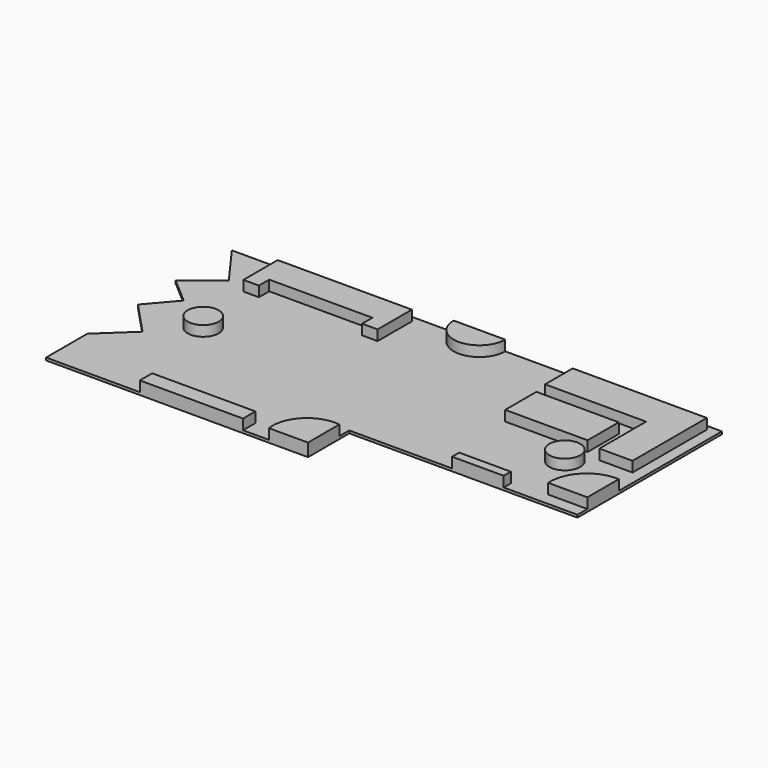
from build123d import *

# Parameters (mm, degrees)
F0_W      = 5077.0874023438
F0_H      = 1000
F1_DEPTH  = 50
F2_W      = 300
F2_H      = 250
F2_W_2    = 1596.8501567841
F2_H_2    = 755.4990053177
F2_W_3    = 1000
F2_H_3    = 172.0993051472
F2_W_4    = 2000
F2_H_4    = 300
F2_R      = 300
F3_DEPTH  = 200
F4_DEPTH  = 200
F5_DEPTH  = 200
F6_DEPTH  = 200
F7_DEPTH  = 200
F8_DEPTH  = 200
F10_DEPTH = 25


# Not quite as in the source:
# - the program builds the solid bodies; features that only make, move or delete a surface that nothing else refers to are left out


with BuildPart() as f1:
    # F0 (on Top) → F1 (new body)
    with BuildSketch(Plane.XY):
        Polygon((-777.0874023438, 2275.4955291748), (-5077.0874023438, 2275.4955291748), (-4499.191295666, 1480.7769234966), (-5119.9254926672, 968.8577861197), (-4616.2895248949, 535.3893431642), (-5077.0874023438, 0), (-4466.0972264549, -651.5435160618), (-5077.0874023438, -1224.5044708252), (0, -1224.5044708252), (4422.9125976562, -1224.5044708252), (4422.9125976562, 2275.4955291748), (222.9125976562, 2275.4955291748), align=None)
        with Locations((-2538.5437011719, -1724.5044708252)):
            Rectangle(F0_W, F0_H)
    extrude(amount=F1_DEPTH)

    # F2 (on face) → F3 (join)
    with BuildSketch(Plane.XY.offset(50)):
        Polygon((-1494.8213815689, 2159.7741413116), (-4094.8213815689, 2159.7741413116), (-4094.8213815689, 1579.7741413116), (-3794.8213815689, 1579.7741413116), (-1794.8213815689, 1579.7741413116), (-1494.8213815689, 1579.7741413116), align=None)
        with Locations((-3944.8213815689, 1454.7741413116)):
            Rectangle(F2_W, F2_H)
        with Locations((-1644.8213815689, 1454.7741413116)):
            Rectangle(F2_W, F2_H)
        Polygon((4209.393954277, 2177.0670413971), (1609.393954277, 2177.0670413971), (1609.393954277, 1507.4201822281), (3566.8230056763, 1507.4201822281), (3566.8230056763, 377.0670413971), (4209.393954277, 377.0670413971), align=None)
        with Locations((2459.3304395676, 854.9439311028)):
            Rectangle(F2_W_2, F2_H_2)
        with Locations((2492.1946525574, -1138.4548182516)):
            Rectangle(F2_W_3, F2_H_3)
        with BuildLine():
            Line((222.9125976562, 2275.4955291748), (-777.0874023438, 2275.4955291748))
            ThreePointArc((-777.0874023438, 2275.4955291748), (-277.0874023438, 1775.4955291748), (222.9125976562, 2275.4955291748))
        make_face()
        with BuildLine():
            Line((3662.9125976562, -984.1235280037), (4422.9125976562, -984.1235280037))
            Line((4422.9125976562, -984.1235280037), (4422.9125976562, -224.1235280037))
            ThreePointArc((4422.9125976562, -224.1235280037), (3868.7706575404, -429.9815878879), (3662.9125976562, -984.1235280037))
        make_face()
        with Locations((-2260, -2074.5044708252)):
            Rectangle(F2_W_4, F2_H_4)
        with BuildLine():
            Line((-760, -2224.5044708252), (0, -2224.5044708252))
            Line((0, -2224.5044708252), (0, -1464.5044708252))
            ThreePointArc((0, -1464.5044708252), (-569.1431166961, -1655.361354129), (-760, -2224.5044708252))
        make_face()
        with Locations((-3832.0874023438, 25.4955291748)):
            Circle(F2_R)
        with Locations((3177.9125976562, 25.4955291748)):
            Circle(F2_R)
    extrude(amount=F3_DEPTH)

    # F2 (on face) → F4 (join)
    with BuildSketch(Plane.XY.offset(50)):
        Polygon((-1494.8213815689, 2159.7741413116), (-4094.8213815689, 2159.7741413116), (-4094.8213815689, 1579.7741413116), (-3794.8213815689, 1579.7741413116), (-1794.8213815689, 1579.7741413116), (-1494.8213815689, 1579.7741413116), align=None)
        with Locations((-3944.8213815689, 1454.7741413116)):
            Rectangle(F2_W, F2_H)
        with Locations((-1644.8213815689, 1454.7741413116)):
            Rectangle(F2_W, F2_H)
        Polygon((4209.393954277, 2177.0670413971), (1609.393954277, 2177.0670413971), (1609.393954277, 1507.4201822281), (3566.8230056763, 1507.4201822281), (3566.8230056763, 377.0670413971), (4209.393954277, 377.0670413971), align=None)
        with Locations((2459.3304395676, 854.9439311028)):
            Rectangle(F2_W_2, F2_H_2)
        with Locations((2492.1946525574, -1138.4548182516)):
            Rectangle(F2_W_3, F2_H_3)
        with BuildLine():
            Line((222.9125976562, 2275.4955291748), (-777.0874023438, 2275.4955291748))
            ThreePointArc((-777.0874023438, 2275.4955291748), (-277.0874023438, 1775.4955291748), (222.9125976562, 2275.4955291748))
        make_face()
        with BuildLine():
            Line((3662.9125976562, -984.1235280037), (4422.9125976562, -984.1235280037))
            Line((4422.9125976562, -984.1235280037), (4422.9125976562, -224.1235280037))
            ThreePointArc((4422.9125976562, -224.1235280037), (3868.7706575404, -429.9815878879), (3662.9125976562, -984.1235280037))
        make_face()
        with Locations((-2260, -2074.5044708252)):
            Rectangle(F2_W_4, F2_H_4)
        with BuildLine():
            Line((-760, -2224.5044708252), (0, -2224.5044708252))
            Line((0, -2224.5044708252), (0, -1464.5044708252))
            ThreePointArc((0, -1464.5044708252), (-569.1431166961, -1655.361354129), (-760, -2224.5044708252))
        make_face()
        with Locations((-3832.0874023438, 25.4955291748)):
            Circle(F2_R)
        with Locations((3177.9125976562, 25.4955291748)):
            Circle(F2_R)
    extrude(amount=F4_DEPTH)

    # F2 (on face) → F5 (join)
    with BuildSketch(Plane.XY.offset(50)):
        Polygon((-1494.8213815689, 2159.7741413116), (-4094.8213815689, 2159.7741413116), (-4094.8213815689, 1579.7741413116), (-3794.8213815689, 1579.7741413116), (-1794.8213815689, 1579.7741413116), (-1494.8213815689, 1579.7741413116), align=None)
        with Locations((-3944.8213815689, 1454.7741413116)):
            Rectangle(F2_W, F2_H)
        with Locations((-1644.8213815689, 1454.7741413116)):
            Rectangle(F2_W, F2_H)
        Polygon((4209.393954277, 2177.0670413971), (1609.393954277, 2177.0670413971), (1609.393954277, 1507.4201822281), (3566.8230056763, 1507.4201822281), (3566.8230056763, 377.0670413971), (4209.393954277, 377.0670413971), align=None)
        with Locations((2459.3304395676, 854.9439311028)):
            Rectangle(F2_W_2, F2_H_2)
        with Locations((2492.1946525574, -1138.4548182516)):
            Rectangle(F2_W_3, F2_H_3)
        with BuildLine():
            Line((222.9125976562, 2275.4955291748), (-777.0874023438, 2275.4955291748))
            ThreePointArc((-777.0874023438, 2275.4955291748), (-277.0874023438, 1775.4955291748), (222.9125976562, 2275.4955291748))
        make_face()
        with BuildLine():
            Line((3662.9125976562, -984.1235280037), (4422.9125976562, -984.1235280037))
            Line((4422.9125976562, -984.1235280037), (4422.9125976562, -224.1235280037))
            ThreePointArc((4422.9125976562, -224.1235280037), (3868.7706575404, -429.9815878879), (3662.9125976562, -984.1235280037))
        make_face()
        with Locations((-2260, -2074.5044708252)):
            Rectangle(F2_W_4, F2_H_4)
        with BuildLine():
            Line((-760, -2224.5044708252), (0, -2224.5044708252))
            Line((0, -2224.5044708252), (0, -1464.5044708252))
            ThreePointArc((0, -1464.5044708252), (-569.1431166961, -1655.361354129), (-760, -2224.5044708252))
        make_face()
        with Locations((-3832.0874023438, 25.4955291748)):
            Circle(F2_R)
        with Locations((3177.9125976562, 25.4955291748)):
            Circle(F2_R)
    extrude(amount=F5_DEPTH)

    # F2 (on face) → F6 (join)
    with BuildSketch(Plane.XY.offset(50)):
        Polygon((-1494.8213815689, 2159.7741413116), (-4094.8213815689, 2159.7741413116), (-4094.8213815689, 1579.7741413116), (-3794.8213815689, 1579.7741413116), (-1794.8213815689, 1579.7741413116), (-1494.8213815689, 1579.7741413116), align=None)
        with Locations((-3944.8213815689, 1454.7741413116)):
            Rectangle(F2_W, F2_H)
        with Locations((-1644.8213815689, 1454.7741413116)):
            Rectangle(F2_W, F2_H)
        Polygon((4209.393954277, 2177.0670413971), (1609.393954277, 2177.0670413971), (1609.393954277, 1507.4201822281), (3566.8230056763, 1507.4201822281), (3566.8230056763, 377.0670413971), (4209.393954277, 377.0670413971), align=None)
        with Locations((2459.3304395676, 854.9439311028)):
            Rectangle(F2_W_2, F2_H_2)
        with Locations((2492.1946525574, -1138.4548182516)):
            Rectangle(F2_W_3, F2_H_3)
        with BuildLine():
            Line((222.9125976562, 2275.4955291748), (-777.0874023438, 2275.4955291748))
            ThreePointArc((-777.0874023438, 2275.4955291748), (-277.0874023438, 1775.4955291748), (222.9125976562, 2275.4955291748))
        make_face()
        with BuildLine():
            Line((3662.9125976562, -984.1235280037), (4422.9125976562, -984.1235280037))
            Line((4422.9125976562, -984.1235280037), (4422.9125976562, -224.1235280037))
            ThreePointArc((4422.9125976562, -224.1235280037), (3868.7706575404, -429.9815878879), (3662.9125976562, -984.1235280037))
        make_face()
        with Locations((-2260, -2074.5044708252)):
            Rectangle(F2_W_4, F2_H_4)
        with BuildLine():
            Line((-760, -2224.5044708252), (0, -2224.5044708252))
            Line((0, -2224.5044708252), (0, -1464.5044708252))
            ThreePointArc((0, -1464.5044708252), (-569.1431166961, -1655.361354129), (-760, -2224.5044708252))
        make_face()
        with Locations((-3832.0874023438, 25.4955291748)):
            Circle(F2_R)
        with Locations((3177.9125976562, 25.4955291748)):
            Circle(F2_R)
    extrude(amount=F6_DEPTH)

    # F2 (on face) → F7 (join)
    with BuildSketch(Plane.XY.offset(50)):
        Polygon((-1494.8213815689, 2159.7741413116), (-4094.8213815689, 2159.7741413116), (-4094.8213815689, 1579.7741413116), (-3794.8213815689, 1579.7741413116), (-1794.8213815689, 1579.7741413116), (-1494.8213815689, 1579.7741413116), align=None)
        with Locations((-3944.8213815689, 1454.7741413116)):
            Rectangle(F2_W, F2_H)
        with Locations((-1644.8213815689, 1454.7741413116)):
            Rectangle(F2_W, F2_H)
        Polygon((4209.393954277, 2177.0670413971), (1609.393954277, 2177.0670413971), (1609.393954277, 1507.4201822281), (3566.8230056763, 1507.4201822281), (3566.8230056763, 377.0670413971), (4209.393954277, 377.0670413971), align=None)
        with Locations((2459.3304395676, 854.9439311028)):
            Rectangle(F2_W_2, F2_H_2)
        with Locations((2492.1946525574, -1138.4548182516)):
            Rectangle(F2_W_3, F2_H_3)
        with BuildLine():
            Line((222.9125976562, 2275.4955291748), (-777.0874023438, 2275.4955291748))
            ThreePointArc((-777.0874023438, 2275.4955291748), (-277.0874023438, 1775.4955291748), (222.9125976562, 2275.4955291748))
        make_face()
        with BuildLine():
            Line((3662.9125976562, -984.1235280037), (4422.9125976562, -984.1235280037))
            Line((4422.9125976562, -984.1235280037), (4422.9125976562, -224.1235280037))
            ThreePointArc((4422.9125976562, -224.1235280037), (3868.7706575404, -429.9815878879), (3662.9125976562, -984.1235280037))
        make_face()
        with Locations((-2260, -2074.5044708252)):
            Rectangle(F2_W_4, F2_H_4)
        with BuildLine():
            Line((-760, -2224.5044708252), (0, -2224.5044708252))
            Line((0, -2224.5044708252), (0, -1464.5044708252))
            ThreePointArc((0, -1464.5044708252), (-569.1431166961, -1655.361354129), (-760, -2224.5044708252))
        make_face()
        with Locations((-3832.0874023438, 25.4955291748)):
            Circle(F2_R)
        with Locations((3177.9125976562, 25.4955291748)):
            Circle(F2_R)
    extrude(amount=F7_DEPTH)

    # F2 (on face) → F8 (join)
    with BuildSketch(Plane.XY.offset(50)):
        Polygon((-1494.8213815689, 2159.7741413116), (-4094.8213815689, 2159.7741413116), (-4094.8213815689, 1579.7741413116), (-3794.8213815689, 1579.7741413116), (-1794.8213815689, 1579.7741413116), (-1494.8213815689, 1579.7741413116), align=None)
        with Locations((-3944.8213815689, 1454.7741413116)):
            Rectangle(F2_W, F2_H)
        with Locations((-1644.8213815689, 1454.7741413116)):
            Rectangle(F2_W, F2_H)
        Polygon((4209.393954277, 2177.0670413971), (1609.393954277, 2177.0670413971), (1609.393954277, 1507.4201822281), (3566.8230056763, 1507.4201822281), (3566.8230056763, 377.0670413971), (4209.393954277, 377.0670413971), align=None)
        with Locations((2459.3304395676, 854.9439311028)):
            Rectangle(F2_W_2, F2_H_2)
        with Locations((2492.1946525574, -1138.4548182516)):
            Rectangle(F2_W_3, F2_H_3)
        with BuildLine():
            Line((222.9125976562, 2275.4955291748), (-777.0874023438, 2275.4955291748))
            ThreePointArc((-777.0874023438, 2275.4955291748), (-277.0874023438, 1775.4955291748), (222.9125976562, 2275.4955291748))
        make_face()
        with BuildLine():
            Line((3662.9125976562, -984.1235280037), (4422.9125976562, -984.1235280037))
            Line((4422.9125976562, -984.1235280037), (4422.9125976562, -224.1235280037))
            ThreePointArc((4422.9125976562, -224.1235280037), (3868.7706575404, -429.9815878879), (3662.9125976562, -984.1235280037))
        make_face()
        with Locations((-2260, -2074.5044708252)):
            Rectangle(F2_W_4, F2_H_4)
        with BuildLine():
            Line((-760, -2224.5044708252), (0, -2224.5044708252))
            Line((0, -2224.5044708252), (0, -1464.5044708252))
            ThreePointArc((0, -1464.5044708252), (-569.1431166961, -1655.361354129), (-760, -2224.5044708252))
        make_face()
        with Locations((-3832.0874023438, 25.4955291748)):
            Circle(F2_R)
        with Locations((3177.9125976562, 25.4955291748)):
            Circle(F2_R)
    extrude(amount=F8_DEPTH)

    # F2 (on face) → F10 (join)
    with BuildSketch(Plane.XY.offset(50)):
        Polygon((-1494.8213815689, 2159.7741413116), (-4094.8213815689, 2159.7741413116), (-4094.8213815689, 1579.7741413116), (-3794.8213815689, 1579.7741413116), (-1794.8213815689, 1579.7741413116), (-1494.8213815689, 1579.7741413116), align=None)
        with Locations((-3944.8213815689, 1454.7741413116)):
            Rectangle(F2_W, F2_H)
        with Locations((-1644.8213815689, 1454.7741413116)):
            Rectangle(F2_W, F2_H)
        Polygon((4209.393954277, 2177.0670413971), (1609.393954277, 2177.0670413971), (1609.393954277, 1507.4201822281), (3566.8230056763, 1507.4201822281), (3566.8230056763, 377.0670413971), (4209.393954277, 377.0670413971), align=None)
        with Locations((2459.3304395676, 854.9439311028)):
            Rectangle(F2_W_2, F2_H_2)
        with Locations((2492.1946525574, -1138.4548182516)):
            Rectangle(F2_W_3, F2_H_3)
        with BuildLine():
            Line((222.9125976562, 2275.4955291748), (-777.0874023438, 2275.4955291748))
            ThreePointArc((-777.0874023438, 2275.4955291748), (-277.0874023438, 1775.4955291748), (222.9125976562, 2275.4955291748))
        make_face()
        with BuildLine():
            Line((3662.9125976562, -984.1235280037), (4422.9125976562, -984.1235280037))
            Line((4422.9125976562, -984.1235280037), (4422.9125976562, -224.1235280037))
            ThreePointArc((4422.9125976562, -224.1235280037), (3868.7706575404, -429.9815878879), (3662.9125976562, -984.1235280037))
        make_face()
        with Locations((-2260, -2074.5044708252)):
            Rectangle(F2_W_4, F2_H_4)
        with BuildLine():
            Line((-760, -2224.5044708252), (0, -2224.5044708252))
            Line((0, -2224.5044708252), (0, -1464.5044708252))
            ThreePointArc((0, -1464.5044708252), (-569.1431166961, -1655.361354129), (-760, -2224.5044708252))
        make_face()
        with Locations((-3832.0874023438, 25.4955291748)):
            Circle(F2_R)
        with Locations((3177.9125976562, 25.4955291748)):
            Circle(F2_R)
    extrude(amount=F10_DEPTH)


solid = f1.part
